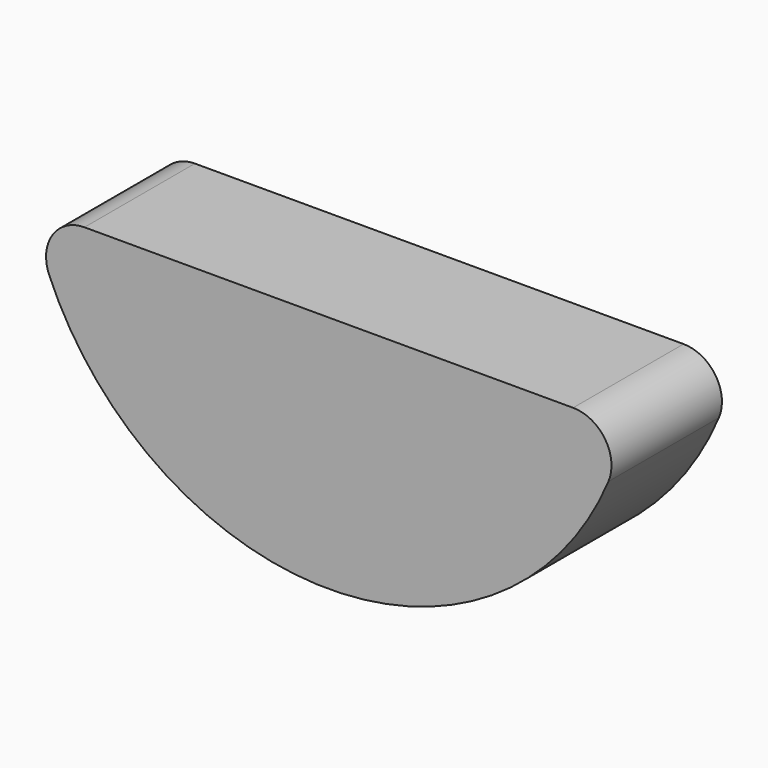
from build123d import *

# Parameters (mm, degrees)
F1_DEPTH = 2.032
F2_R     = 1.1303


with BuildPart() as f1:
    # F0 (on Front) → F1 (new body, symmetric)
    with BuildSketch(Plane.XZ):
        with BuildLine():
            Line((8.5769976952, 0), (-8.8855023048, 0))
            ThreePointArc((-8.8855023048, 0), (-0.1542523048, -7.0358), (8.5769976952, 0))
        make_face()
    extrude(amount=F1_DEPTH, both=True)

    # F2
    f2_edges = [f1.edges().sort_by_distance(p)[0] for p in [
        (-8.885502, 0, 0),
        (8.576998, 0, 0),
    ]]
    fillet(f2_edges, radius=F2_R)


solid = f1.part
